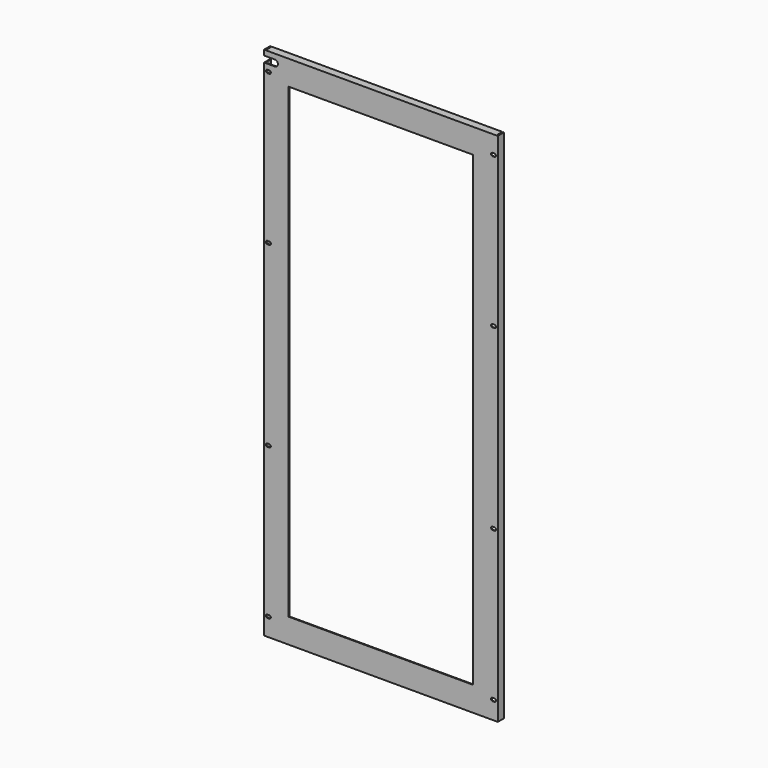
from build123d import *

# Parameters (mm, degrees)
F0_W              = 482.6
F0_H              = 1065.2125
F1_DEPTH          = 1.6
F2_W              = 15.875
F2_H              = 1065.2125
F3_DEPTH          = 1.6
F4_W              = 15.875
F4_H              = 1065.2125
F5_DEPTH          = 1.6
F6_W              = 476.25
F6_H              = 15.875
F7_DEPTH          = 1.6
F8_W              = 476.25
F8_H              = 15.875
F9_DEPTH          = 1.6
F10_W             = 381
F10_H             = 963.6125
F11_DEPTH         = 1.6
F12_W             = 3.96875
F12_H             = 6.35
F13_DEPTH         = 1.6
F13_COPIES3_COUNT = 2
F13_COPIES3_PITCH = 1094.309536
F13_COPIES4_COUNT = 2
F13_COPIES4_PITCH = 823.333045
F14_W             = 3.96875
F14_H             = 6.35
F15_DEPTH         = 1.6
F16_W             = 22.225
F16_H             = 12.7
F17_DEPTH         = 16


# Not quite as in the source:
# - a pattern or mirror of a feature is missing from the dataset's text; its kind, count and spacing are read off the source's solid


with BuildPart() as f1:
    # F0 (on Front) → F1 (new body)
    with BuildSketch(Plane.XZ):
        Rectangle(F0_W, F0_H)
    extrude(amount=-F1_DEPTH)

    # F2 (on face) → F3 (join)
    with BuildSketch(Plane(origin=(-241.3, 0, 0), x_dir=(0, -1, 0), z_dir=(-1, 0, 0))):
        with Locations((-7.9375, 0)):
            Rectangle(F2_W, F2_H)
    extrude(amount=-F3_DEPTH)

    # F4 (on face) → F5 (join)
    with BuildSketch(Plane.YZ.offset(241.3)):
        with Locations((7.9375, 0)):
            Rectangle(F4_W, F4_H)
    extrude(amount=-F5_DEPTH)

    # F6 (on face) → F7 (join)
    with BuildSketch(Plane.XY.offset(532.60625)):
        with Locations((0, 7.9375)):
            Rectangle(F6_W, F6_H)
    extrude(amount=-F7_DEPTH)

    # F8 (on face) → F9 (join)
    with BuildSketch(Plane(origin=(0, 0, -532.60625), x_dir=(1, 0, 0), z_dir=(0, 0, -1))):
        with Locations((0, -7.9375)):
            Rectangle(F8_W, F8_H)
    extrude(amount=-F9_DEPTH)

    # F10 (on face) → F11 (cut)
    with BuildSketch(Plane.XZ):
        Rectangle(F10_W, F10_H)
    extrude(amount=-F11_DEPTH, mode=Mode.SUBTRACT)

    # F12 (on face) → F13 (cut)
    with BuildSketch(Plane.XZ):
        with Locations((-232.5, -495.3)):
            Rectangle(F12_W, F12_H)
        with BuildLine():
            Line((-230.515625, -492.125), (-230.515625, -498.475))
            ThreePointArc((-230.515625, -498.475), (-227.340625, -495.3), (-230.515625, -492.125))
        make_face()
        with BuildLine():
            ThreePointArc((-234.484375, -492.125), (-237.659375, -495.3), (-234.484375, -498.475))
            Line((-234.484375, -498.475), (-234.484375, -492.125))
        make_face()
    f13 = extrude(amount=-F13_DEPTH, mode=Mode.SUBTRACT)

    # F13_copies: F13 across plane
    add(f13.mirror(Plane.XY), mode=Mode.SUBTRACT)

    # F13_copies1: F13 across plane
    add(f13.mirror(Plane.XY.offset(-155.575)), mode=Mode.SUBTRACT)

    # F13_copies2: F13 across plane
    add(f13.mirror(Plane(origin=(0, 0, 0), x_dir=(0, 0, 1), z_dir=(1, 0, 0))), mode=Mode.SUBTRACT)

    # F13_copies3: F13 ×2
    with Locations(*[Vector(0.4249254757, 0, 0.9052283359) * (i * F13_COPIES3_PITCH) for i in range(1, F13_COPIES3_COUNT)]):
        add(f13, mode=Mode.SUBTRACT)

    # F13_copies4: F13 ×2
    with Locations(*[Vector(0.5647775259, 0, 0.8252432043) * (i * F13_COPIES4_PITCH) for i in range(1, F13_COPIES4_COUNT)]):
        add(f13, mode=Mode.SUBTRACT)

    # F14 (on face) → F15 (cut)
    with BuildSketch(Plane.XZ):
        with Locations((-232.5, -184.15)):
            Rectangle(F14_W, F14_H)
        with BuildLine():
            Line((-230.515625, -180.975), (-230.515625, -187.325))
            ThreePointArc((-230.515625, -187.325), (-227.340625, -184.15), (-230.515625, -180.975))
        make_face()
        with BuildLine():
            ThreePointArc((-234.484375, -180.975), (-237.659375, -184.15), (-234.484375, -187.325))
            Line((-234.484375, -187.325), (-234.484375, -180.975))
        make_face()
    f15 = extrude(amount=-F15_DEPTH, mode=Mode.SUBTRACT)

    # F15_copies: F15 across plane
    add(f15.mirror(Plane(origin=(0, 0, 0), x_dir=(0, 0, 1), z_dir=(1, 0, 0))), mode=Mode.SUBTRACT)

    # F16 (on face) → F17 (cut)
    with BuildSketch(Plane.XZ):
        with Locations((-230.1875, 515.540625)):
            Rectangle(F16_W, F16_H)
        with BuildLine():
            Line((-219.075, 521.890625), (-219.075, 509.190625))
            ThreePointArc((-219.075, 509.190625), (-212.725, 515.540625), (-219.075, 521.890625))
        make_face()
    extrude(amount=-F17_DEPTH, mode=Mode.SUBTRACT)


solid = f1.part
